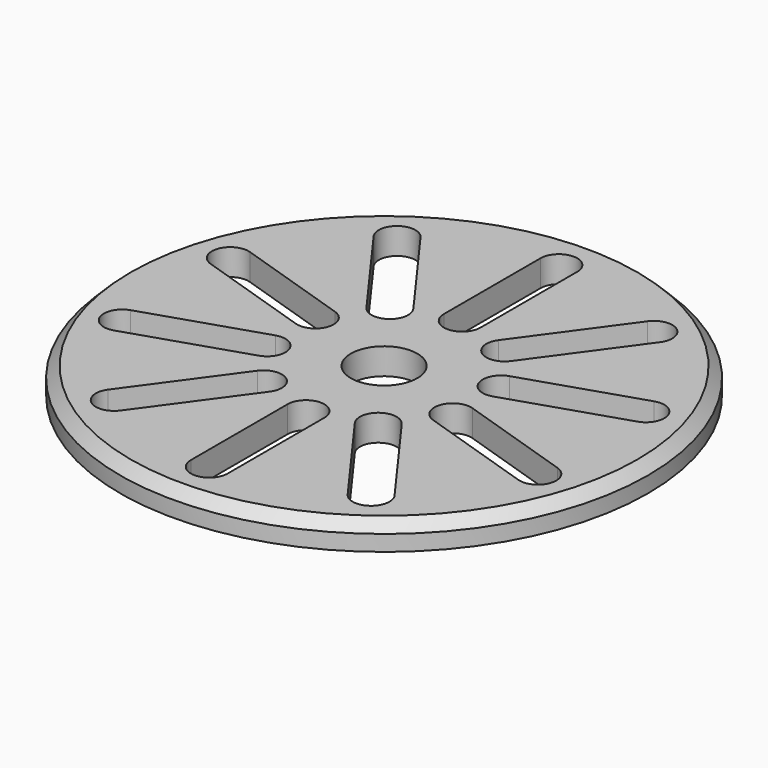
from build123d import *

# Parameters (mm, degrees)
F0_R     = 63.5
F0_R_2   = 12.7
F1_DEPTH = 6.35
F2_T     = 5.08
F3_SIZE  = 2.54
F4_R     = 12.7
F4_R_2   = 8.001
F5_DEPTH = 6.35


# Not quite as in the source:
# - a shell that OpenCascade refuses in one call is made with other operations: the cavity is built on its own and cut out


with BuildPart() as f1:
    # F0 (on Top) → F1 (new body)
    with BuildSketch(Plane.XY):
        Circle(F0_R)
        with BuildLine():
            ThreePointArc((4.4125195695, -52.5690356897), (0, -56.9815552592), (-4.4125195695, -52.5690356897))
            Line((-4.4125195695, -52.5690356897), (-4.4125195695, -23.4904065728))
            ThreePointArc((-4.4125195695, -23.4904065728), (0, -19.0778870033), (4.4125195695, -23.4904065728))
            Line((4.4125195695, -23.4904065728), (4.4125195695, -52.5690356897))
        make_face(mode=Mode.SUBTRACT)
        with BuildLine():
            ThreePointArc((-48.6325804131, -20.4412808959), (-54.1926794379, -17.608268941), (-51.359667483, -12.0481699162))
            Line((-51.359667483, -12.0481699162), (-23.7042477765, -3.0623793459))
            ThreePointArc((-23.7042477765, -3.0623793459), (-18.1441487516, -5.8953913008), (-20.9771607065, -11.4554903256))
            Line((-20.9771607065, -11.4554903256), (-48.6325804131, -20.4412808959))
        make_face(mode=Mode.SUBTRACT)
        with BuildLine():
            ThreePointArc((-27.3295005859, -45.1228571793), (-33.4929178341, -46.0990465706), (-34.4691072254, -39.9356293225))
            Line((-34.4691072254, -39.9356293225), (-17.3771178736, -16.4105241938))
            ThreePointArc((-17.3771178736, -16.4105241938), (-11.2137006254, -15.4343348024), (-10.2375112341, -21.5977520506))
            Line((-10.2375112341, -21.5977520506), (-27.3295005859, -45.1228571793))
        make_face(mode=Mode.SUBTRACT)
        with BuildLine():
            ThreePointArc((34.4691072254, -39.9356293225), (33.4929178341, -46.0990465706), (27.3295005859, -45.1228571793))
            Line((27.3295005859, -45.1228571793), (10.2375112341, -21.5977520506))
            ThreePointArc((10.2375112341, -21.5977520506), (11.2137006254, -15.4343348024), (17.3771178736, -16.4105241938))
            Line((17.3771178736, -16.4105241938), (34.4691072254, -39.9356293225))
        make_face(mode=Mode.SUBTRACT)
        with BuildLine():
            ThreePointArc((51.359667483, -12.0481699162), (54.1926794379, -17.608268941), (48.6325804131, -20.4412808959))
            Line((48.6325804131, -20.4412808959), (20.9771607065, -11.4554903256))
            ThreePointArc((20.9771607065, -11.4554903256), (18.1441487516, -5.8953913008), (23.7042477765, -3.0623793459))
            Line((23.7042477765, -3.0623793459), (51.359667483, -12.0481699162))
        make_face(mode=Mode.SUBTRACT)
        with BuildLine():
            ThreePointArc((-51.359667483, 12.0481699162), (-54.1926794379, 17.608268941), (-48.6325804131, 20.4412808959))
            Line((-48.6325804131, 20.4412808959), (-20.9771607065, 11.4554903256))
            ThreePointArc((-20.9771607065, 11.4554903256), (-18.1441487516, 5.8953913008), (-23.7042477765, 3.0623793459))
            Line((-23.7042477765, 3.0623793459), (-51.359667483, 12.0481699162))
        make_face(mode=Mode.SUBTRACT)
        with BuildLine():
            ThreePointArc((-34.4691072254, 39.9356293225), (-33.4929178341, 46.0990465706), (-27.3295005859, 45.1228571793))
            Line((-27.3295005859, 45.1228571793), (-10.2375112341, 21.5977520506))
            ThreePointArc((-10.2375112341, 21.5977520506), (-11.2137006254, 15.4343348024), (-17.3771178736, 16.4105241938))
            Line((-17.3771178736, 16.4105241938), (-34.4691072254, 39.9356293225))
        make_face(mode=Mode.SUBTRACT)
        Circle(F0_R_2, mode=Mode.SUBTRACT)
        with BuildLine():
            ThreePointArc((27.3295005859, 45.1228571793), (33.4929178341, 46.0990465706), (34.4691072254, 39.9356293225))
            Line((34.4691072254, 39.9356293225), (17.3771178736, 16.4105241938))
            ThreePointArc((17.3771178736, 16.4105241938), (11.2137006254, 15.4343348024), (10.2375112341, 21.5977520506))
            Line((10.2375112341, 21.5977520506), (27.3295005859, 45.1228571793))
        make_face(mode=Mode.SUBTRACT)
        with BuildLine():
            ThreePointArc((48.6325804131, 20.4412808959), (54.1926794379, 17.608268941), (51.359667483, 12.0481699162))
            Line((51.359667483, 12.0481699162), (23.7042477765, 3.0623793459))
            ThreePointArc((23.7042477765, 3.0623793459), (18.1441487516, 5.8953913008), (20.9771607065, 11.4554903256))
            Line((20.9771607065, 11.4554903256), (48.6325804131, 20.4412808959))
        make_face(mode=Mode.SUBTRACT)
        with BuildLine():
            Line((4.4125195695, 52.5690356897), (4.4125195695, 23.4904065728))
            ThreePointArc((4.4125195695, 23.4904065728), (0, 19.0778870033), (-4.4125195695, 23.4904065728))
            Line((-4.4125195695, 23.4904065728), (-4.4125195695, 52.5690356897))
            ThreePointArc((-4.4125195695, 52.5690356897), (0, 56.9815552592), (4.4125195695, 52.5690356897))
        make_face(mode=Mode.SUBTRACT)
    extrude(amount=F1_DEPTH)

    # F2: shell of thickness 5.08, made by hand


with BuildPart() as f2_core1:
    # F2_t2: copy of F1
    add(f1.part)

    # the walls: a layer under each face that stays
    f2_faces = [f2_core1.faces().sort_by_distance(p)[0] for p in [
        (-63.5, 0, 3.175),
        (4.4125195695, -38.0297211313, 3.175),
        (0, -56.9815552592, 3.175),
        (-4.4125195695, -38.0297211313, 3.175),
        (0, -19.0778870033, 3.175),
        (-18.1441487516, -5.8953913008, 3.175),
        (-34.8048705598, -15.9483856108, 3.175),
        (-54.1926794379, -17.608268941, 3.175),
        (-37.5319576298, -7.555274631, 3.175),
        (-18.78350591, -33.3603046149, 3.175),
        (-33.4929178341, -46.0990465706, 3.175),
        (-25.9231125495, -28.1730767581, 3.175),
        (-11.2137006254, -15.4343348024, 3.175),
        (11.2137006254, -15.4343348024, 3.175),
        (25.9231125495, -28.1730767581, 3.175),
        (33.4929178341, -46.0990465706, 3.175),
        (18.78350591, -33.3603046149, 3.175),
        (18.1441487516, -5.8953913008, 3.175),
        (37.5319576298, -7.555274631, 3.175),
        (54.1926794379, -17.608268941, 3.175),
        (34.8048705598, -15.9483856108, 3.175),
        (-37.5319576298, 7.555274631, 3.175),
        (-54.1926794379, 17.608268941, 3.175),
        (-34.8048705598, 15.9483856108, 3.175),
        (-18.1441487516, 5.8953913008, 3.175),
        (-25.9231125495, 28.1730767581, 3.175),
        (-33.4929178341, 46.0990465706, 3.175),
        (-18.78350591, 33.3603046149, 3.175),
        (-11.2137006254, 15.4343348024, 3.175),
        (-12.7, 0, 3.175),
        (11.2137006254, 15.4343348024, 3.175),
        (18.78350591, 33.3603046149, 3.175),
        (33.4929178341, 46.0990465706, 3.175),
        (25.9231125495, 28.1730767581, 3.175),
        (18.1441487516, 5.8953913008, 3.175),
        (34.8048705598, 15.9483856108, 3.175),
        (54.1926794379, 17.608268941, 3.175),
        (37.5319576298, 7.555274631, 3.175),
        (0, 19.0778870033, 3.175),
        (-4.4125195695, 38.0297211313, 3.175),
        (0, 56.9815552592, 3.175),
        (4.4125195695, 38.0297211313, 3.175),
        (-42.3333333333, -42.3333333333, 6.35),
    ]]
    thicken(f2_faces, amount=-F2_T, mode=Mode.SUBTRACT)


with BuildPart() as f1_1:
    add(f1.part)

    # what is left inside the walls is the cavity
    f2_cavity = [f2_core1.part.solids().sort_by_distance(p)[0] for p in [
        (17.763773, -48.3307, 1.2192),
        (38.738777, -34.159737, 1.2192),
        (44.569219, -3.470458, 1.2192),
        (38.738777, 26.107791, 1.2192),
        (12.812871, 48.3307, 1.2192),
        (-22.714676, 48.3307, 0.0508),
        (-38.738777, 26.107791, 0.0508),
        (-44.569219, -3.470458, 0.0508),
        (-38.738777, -34.159737, 1.2192),
        (-17.763773, -48.3307, 0.0508),
    ]]
    add(f2_cavity, mode=Mode.SUBTRACT)

    # F3
    f3_edges = [f1_1.edges().sort_by_distance(p)[0] for p in [
        (-63.5, 0, 6.35),
    ]]
    chamfer(f3_edges, length=F3_SIZE)

    # F4 (on face) → F5 (join)
    with BuildSketch(Plane.XY.offset(6.35)):
        Circle(F4_R)
        Circle(F4_R_2, mode=Mode.SUBTRACT)
    extrude(amount=-F5_DEPTH)


solid = f1_1.part
